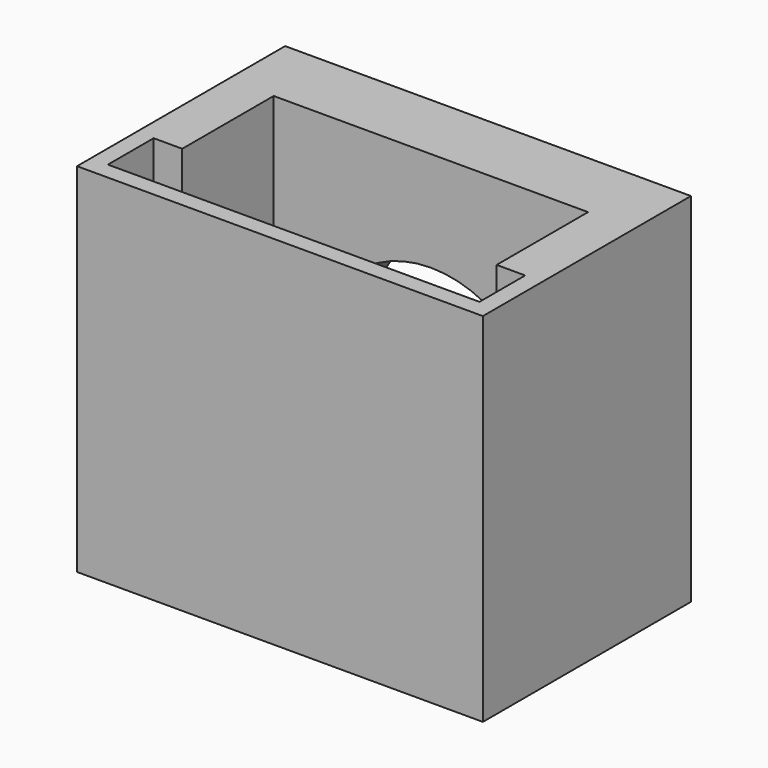
from build123d import *

# Parameters (mm, degrees)
F0_W     = 28.4
F0_H     = 18.2
F1_DEPTH = 25
F0_W_2   = 22
F0_H_2   = 8
F2_DEPTH = 1.2
F3_R     = 8
F4_DEPTH = 5


with BuildPart() as f1:
    # F0 (on Top) → F1 (new body)
    with BuildSketch(Plane.XY):
        with Locations((0, 5.9)):
            Rectangle(F0_W, F0_H)
        Polygon((11, 2), (13, 2), (13, -2), (-13, -2), (-13, 2), (-11, 2), (-11, 10), (11, 10), align=None, mode=Mode.SUBTRACT)
    extrude(amount=F1_DEPTH)

    # F0 (on Top) → F2 (join)
    with BuildSketch(Plane.XY):
        with Locations((0, 6)):
            Rectangle(F0_W_2, F0_H_2)
        Polygon((13, -2), (13, 2), (11, 2), (-11, 2), (-13, 2), (-13, -2), align=None)
    extrude(amount=F2_DEPTH)

    # F3 (on face) → F4 (cut)
    with BuildSketch(Plane(origin=(0, 15, 0), x_dir=(-1, 0, 0), z_dir=(0, 1, 0))):
        with Locations((0, 10)):
            Circle(F3_R)
    extrude(amount=-F4_DEPTH, mode=Mode.SUBTRACT)


solid = f1.part
